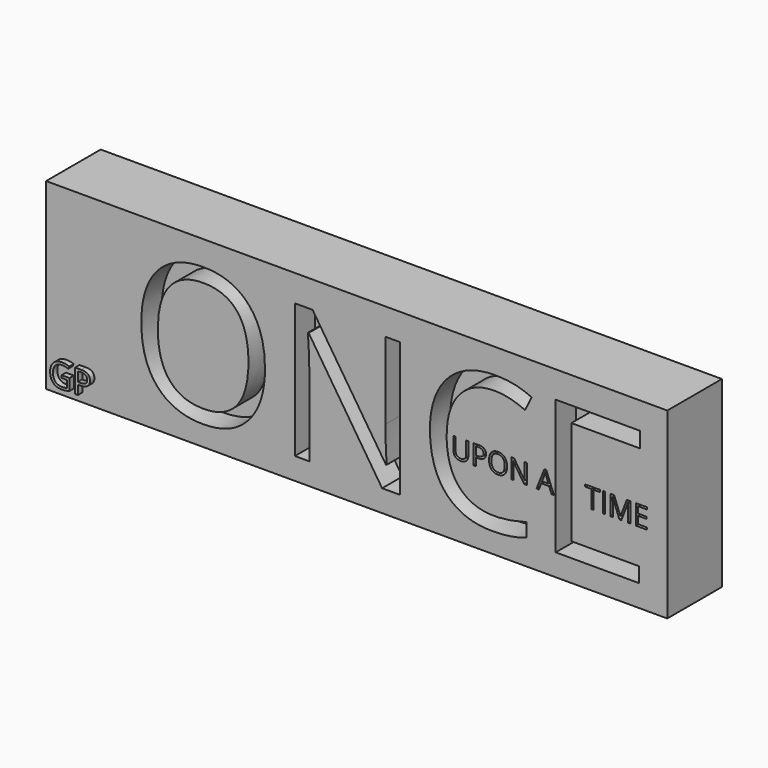
from build123d import *

# Parameters (mm, degrees)
F0_W          = 231.106877327
F0_H          = 68.1117326021
F1_DEPTH      = 25.4
F2_TEXT_SIZE  = 70.057032113
F3_DEPTH      = 9.398
F4_TEXT_SIZE  = 10.2115436734
F5_DEPTH      = 8.636
F6_TEXT_SIZE  = 10.3555839612
F7_DEPTH      = 8.636
F8_W          = 25.618191997
F8_H          = 5.780675191
F8_W_2        = 25.2151602901
F8_H_2        = 5.5427953904
F9_DEPTH      = 9.398
F10_TEXT_SIZE = 12.1879029191
F11_DEPTH     = 2.032


# Not quite as in the source:
# - Text() gives the source's letters only with a copy of the font that has no kerning and outlines rounded to 1/6400 em; it was checked with that copy


with BuildPart() as f1:
    # F0 (on Front) → F1 (new body)
    with BuildSketch(Plane.XZ):
        Rectangle(F0_W, F0_H)
    extrude(amount=F1_DEPTH)

    # F2 (on face) → F3 (cut)
    with BuildSketch(Plane.XZ.offset(25.4)):
        with Locations((-84.4023040793, -25.8957103198)):
            Text('ONCI', F2_TEXT_SIZE, font='Open Sans', text_align=(TextAlign.LEFT, TextAlign.BOTTOM))
    extrude(amount=-F3_DEPTH, mode=Mode.SUBTRACT)

    # F4 (on face) → F5 (cut)
    with BuildSketch(Plane.XZ.offset(25.4)):
        with Locations((35.0373066341, -7.3523114448)):
            Text('UPON A', F4_TEXT_SIZE, font='Open Sans', text_align=(TextAlign.LEFT, TextAlign.BOTTOM))
    extrude(amount=-F5_DEPTH, mode=Mode.SUBTRACT)

    # F6 (on face) → F7 (cut)
    with BuildSketch(Plane.XZ.offset(25.4)):
        with Locations((84.8472958322, -7.4560204521)):
            Text('TIME', F6_TEXT_SIZE, font='Open Sans', text_align=(TextAlign.LEFT, TextAlign.BOTTOM))
    extrude(amount=-F7_DEPTH, mode=Mode.SUBTRACT)

    # F8 (on face) → F9 (cut)
    with BuildSketch(Plane.XZ.offset(25.4)):
        with Locations((92.6686394017, 21.2281051667)):
            Rectangle(F8_W, F8_H)
        with Locations((92.4671235483, -23.1243126246)):
            Rectangle(F8_W_2, F8_H_2)
    extrude(amount=-F9_DEPTH, mode=Mode.SUBTRACT)

    # F10 (on face) → F11 (join)
    with BuildSketch(Plane.XZ.offset(25.4)):
        with Locations((-113.1754294038, -30.8425650001)):
            Text('GP', F10_TEXT_SIZE, font='Open Sans', text_align=(TextAlign.LEFT, TextAlign.BOTTOM))
    extrude(amount=F11_DEPTH)


solid = f1.part
